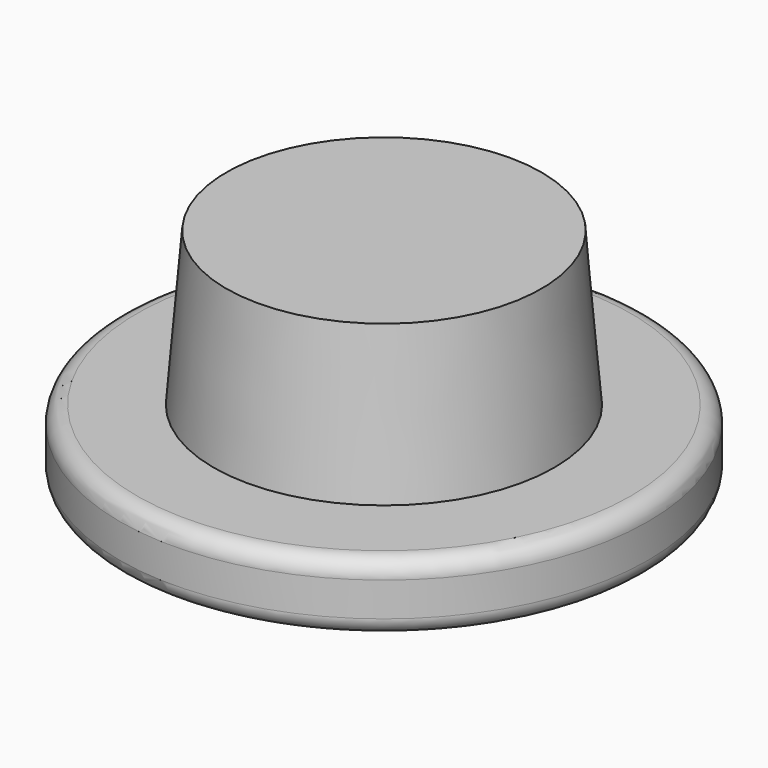
from build123d import *

# Parameters (mm, degrees)
F2_R         = 31
F3_DEPTH     = 8
F4_R         = 2
F5_R         = 2
F6_TEXT_SIZE = 18.3995302197
F7_DEPTH     = 1
F9_ANGLE     = 180


# Not quite as in the source:
# - Text() gives the source's letters only with a copy of the font that has no kerning and outlines rounded to 1/6400 em; it was checked with that copy


with BuildPart() as f1:
    # F0 (on Right) → F1 (revolve)
    with BuildSketch(Plane.YZ):
        Polygon((-18.5, 0), (0, 0), (0, 18), (-20, 18), align=None)
    revolve(axis=Axis((0, 0, 9), (0, 0, 1)))

    # F2 (on face) → F3 (join)
    with BuildSketch(Plane.XY.offset(18)):
        Circle(F2_R)
    extrude(amount=F3_DEPTH)

    # F4
    f4_edges = [f1.edges().sort_by_distance(p)[0] for p in [
        (-31, 0, 26),
    ]]
    fillet(f4_edges, radius=F4_R)

    # F5
    f5_edges = [f1.edges().sort_by_distance(p)[0] for p in [
        (-31, 0, 18),
    ]]
    fillet(f5_edges, radius=F5_R)

    # F6 (on face) → F7 (cut)
    with BuildSketch(Plane.XY.offset(26)):
        with Locations((-28.2180118674, -6.5585806368)):
            Text('Diesel', F6_TEXT_SIZE, font='Open Sans', font_style=FontStyle.BOLD, text_align=(TextAlign.LEFT, TextAlign.BOTTOM))
    extrude(amount=-F7_DEPTH, mode=Mode.SUBTRACT)


with BuildPart() as f1_1:
    # F9: moved
    add(f1.part.rotate(Axis((-1.0011773556, 0, 0), (1, 0, 0)), F9_ANGLE))


solid = f1_1.part
